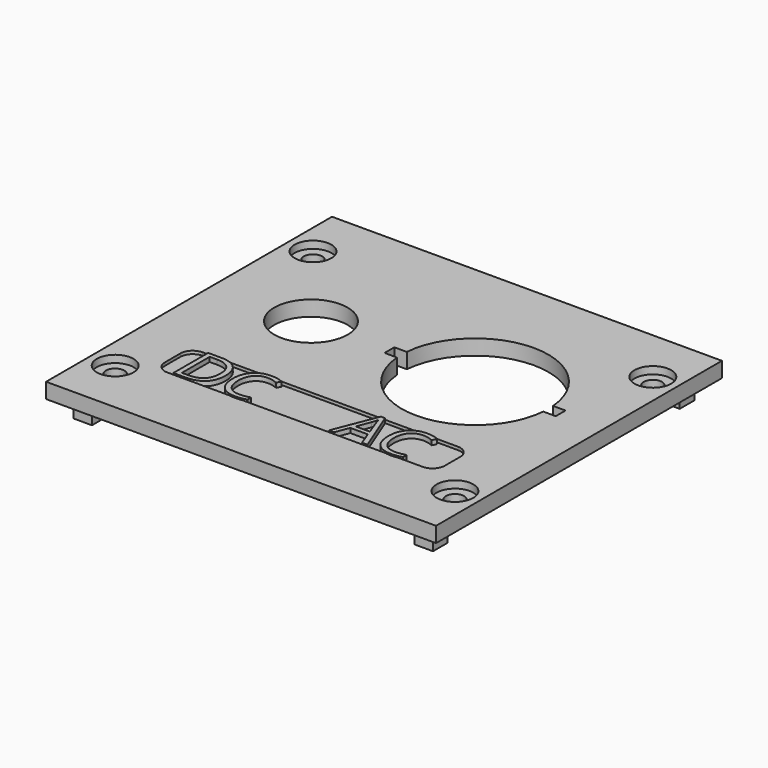
from build123d import *

# Parameters (mm, degrees)
F0_W          = 63.772
F0_H          = 58.442
F1_DEPTH      = 2.5
F2_W          = 58.772
F2_H          = 53.442
F2_W_2        = 54.772
F2_H_2        = 49.442
F3_DEPTH      = 3
F4_W          = 52.772
F4_H          = 2
F5_DEPTH      = 3
F6_W          = 56.772
F6_H          = 47.442
F6_W_2        = 2
F7_DEPTH      = 3
F8_R          = 6
F8_R_2        = 12
F9_DEPTH      = 2.5
F10_W         = 28
F10_H         = 2
F11_DEPTH     = 3
F12_R         = 1.5
F13_DEPTH     = 2.5
F12_R_2       = 3
F14_DEPTH     = 1.25
F15_R         = 3
F15_R_2       = 1.5
F16_DEPTH     = 1.2
F18_DEPTH     = 0.5
F19_TEXT_SIZE = 9.9547854107
F20_DEPTH     = 0.75


# Not quite as in the source:
# - Text() gives the source's letters only with a copy of the font that has no kerning and outlines rounded to 1/6400 em; it was checked with that copy


with BuildPart() as f1:
    # F0 (on Top) → F1 (new body)
    with BuildSketch(Plane.XY):
        Rectangle(F0_W, F0_H)
    extrude(amount=-F1_DEPTH)

    # F2 (on face) → F3 (join)
    with BuildSketch(Plane(origin=(0, 0, -2.5), x_dir=(1, 0, 0), z_dir=(0, 0, -1))):
        Rectangle(F2_W, F2_H)
        Rectangle(F2_W_2, F2_H_2, mode=Mode.SUBTRACT)
    extrude(amount=F3_DEPTH)

    # F4 (on face) → F5 (cut)
    with BuildSketch(Plane(origin=(0, 0, -5.5), x_dir=(1, 0, 0), z_dir=(0, 0, -1))):
        with Locations((0, 25.721)):
            Rectangle(F4_W, F4_H)
        with Locations((0, -25.721)):
            Rectangle(F4_W, F4_H)
    extrude(amount=-F5_DEPTH, mode=Mode.SUBTRACT)

    # F6 (on face) → F7 (cut)
    with BuildSketch(Plane(origin=(0, 0, -5.5), x_dir=(1, 0, 0), z_dir=(0, 0, -1))):
        with Locations((1, 0)):
            Rectangle(F6_W, F6_H)
        with Locations((-28.386, 0)):
            Rectangle(F6_W_2, F6_H)
    extrude(amount=-F7_DEPTH, mode=Mode.SUBTRACT)

    # F8 (on face) → F9 (cut)
    with BuildSketch(Plane.XY):
        with Locations((-15.943, 5)):
            Circle(F8_R)
        with Locations((10.886, 5)):
            Circle(F8_R_2)
    extrude(amount=-F9_DEPTH, mode=Mode.SUBTRACT)

    # F10 (on Top) → F11 (cut)
    with BuildSketch(Plane.XY):
        with Locations((10.886, 5)):
            Rectangle(F10_W, F10_H)
    extrude(amount=-F11_DEPTH, mode=Mode.SUBTRACT)

    # F12 (on face) → F13 (cut)
    with BuildSketch(Plane(origin=(0, 0, -2.5), x_dir=(1, 0, 0), z_dir=(0, 0, -1))):
        with Locations((-27.786, -20.221)):
            Circle(F12_R)
        with Locations((27.786, -20.221)):
            Circle(F12_R)
        with Locations((27.786, 20.221)):
            Circle(F12_R)
        with Locations((-27.786, 20.221)):
            Circle(F12_R)
    extrude(amount=-F13_DEPTH, mode=Mode.SUBTRACT)

    # F12 (on face) → F14 (cut)
    with BuildSketch(Plane(origin=(0, 0, -2.5), x_dir=(1, 0, 0), z_dir=(0, 0, -1))):
        with Locations((-27.786, -20.221)):
            Circle(F12_R_2)
        with Locations((-27.786, -20.221)):
            Circle(F12_R, mode=Mode.SUBTRACT)
        with Locations((27.786, -20.221)):
            Circle(F12_R_2)
        with Locations((27.786, -20.221)):
            Circle(F12_R, mode=Mode.SUBTRACT)
        with Locations((27.786, 20.221)):
            Circle(F12_R_2)
        with Locations((27.786, 20.221)):
            Circle(F12_R, mode=Mode.SUBTRACT)
        with Locations((-27.786, 20.221)):
            Circle(F12_R_2)
        with Locations((-27.786, 20.221)):
            Circle(F12_R, mode=Mode.SUBTRACT)
    extrude(amount=F14_DEPTH, mode=Mode.SUBTRACT)

    # F15 (on face) → F16 (cut)
    with BuildSketch(Plane.XY):
        with Locations((-27.786, 20.221)):
            Circle(F15_R)
        with Locations((-27.786, 20.221)):
            Circle(F15_R_2, mode=Mode.SUBTRACT)
        with Locations((27.786, 20.221)):
            Circle(F15_R)
        with Locations((27.786, 20.221)):
            Circle(F15_R_2, mode=Mode.SUBTRACT)
        with Locations((27.786, -20.221)):
            Circle(F15_R)
        with Locations((27.786, -20.221)):
            Circle(F15_R_2, mode=Mode.SUBTRACT)
        with Locations((-27.786, -20.221)):
            Circle(F15_R)
        with Locations((-27.786, -20.221)):
            Circle(F15_R_2, mode=Mode.SUBTRACT)
    extrude(amount=-F16_DEPTH, mode=Mode.SUBTRACT)

    # F17 (on face) → F18 (cut)
    with BuildSketch(Plane.XY):
        with BuildLine():
            Line((20.386, -10.383605957), (-21.386, -10.383605957))
            ThreePointArc((-21.386, -10.383605957), (-22.8002135624, -10.9693923947), (-23.386, -12.383605957))
            Line((-23.386, -12.383605957), (-23.386, -15.5510514528))
            ThreePointArc((-23.386, -15.5510514528), (-22.8002135624, -16.9652650151), (-21.386, -17.5510514528))
            Line((-21.386, -17.5510514528), (20.386, -17.5510514528))
            ThreePointArc((20.386, -17.5510514528), (21.8002135624, -16.9652650151), (22.386, -15.5510514528))
            Line((22.386, -15.5510514528), (22.386, -12.383605957))
            ThreePointArc((22.386, -12.383605957), (21.8002135624, -10.9693923947), (20.386, -10.383605957))
        make_face()
    extrude(amount=-F18_DEPTH, mode=Mode.SUBTRACT)

    # F19 (on face) → F20 (join)
    with BuildSketch(Plane.XY.offset(-0.5)):
        with Locations((-21.386, -17.5510514528)):
            Text('DC', F19_TEXT_SIZE, font='Open Sans', text_align=(TextAlign.LEFT, TextAlign.BOTTOM))
        with Locations((5.0143948756, -17.5510514528)):
            Text('AC', F19_TEXT_SIZE, font='Open Sans', text_align=(TextAlign.LEFT, TextAlign.BOTTOM))
    extrude(amount=F20_DEPTH)


solid = f1.part
